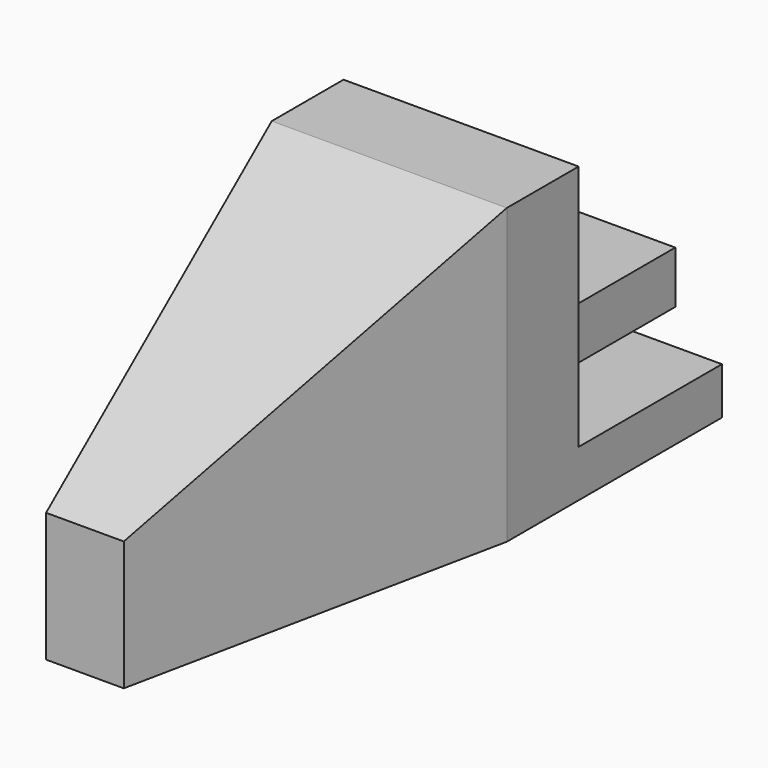
from build123d import *

# Parameters (mm, degrees)
F0_W     = 4.064
F0_H     = 3
F1_DEPTH = 15.24
F2_W     = 20
F2_H     = 25
F3_DEPTH = 40
F5_DEPTH = 25.001
F7_DEPTH = 20.001


# Not quite as in the source:
# - a pattern or mirror of a feature is missing from the dataset's text; its kind, count and spacing are read off the source's solid


with BuildPart() as f1:
    # F0 (on Front) → F1 (new body)
    with BuildSketch(Plane.XZ):
        Polygon((6.0325, 4.445), (-6.0325, 4.445), (-6.0325, 0), (-2.032, 0), (2.032, 0), (6.0325, 0), align=None)
        with Locations((0, -1.5)):
            Rectangle(F0_W, F0_H)
        Polygon((2.032, -3), (-2.032, -3), (-10, -3), (-10, -7), (10, -7), (10, -3), align=None)
    extrude(amount=-F1_DEPTH)

    # F2 (on face) → F3 (join)
    with BuildSketch(Plane.XZ):
        with Locations((0, 5.5)):
            Rectangle(F2_W, F2_H)
    extrude(amount=F3_DEPTH)

    # F4 (on face) → F5 (cut, through all)
    with BuildSketch(Plane.XY.offset(18)):
        Polygon((-3.305207938, -40), (-10, -7.6365470886), (-10, -40), align=None)
    f5 = extrude(amount=-F5_DEPTH, mode=Mode.SUBTRACT)

    # F5_copies: F5 across plane
    add(f5.mirror(Plane(origin=(0, 0, 0), x_dir=(0, 0, 1), z_dir=(1, 0, 0))), mode=Mode.SUBTRACT)

    # F6 (on face) → F7 (cut, through all)
    with BuildSketch(Plane.YZ.offset(10)):
        Polygon((-40, 18), (-40, 4), (-7.6365470886, 18), align=None)
    extrude(amount=-F7_DEPTH, mode=Mode.SUBTRACT)


solid = f1.part
